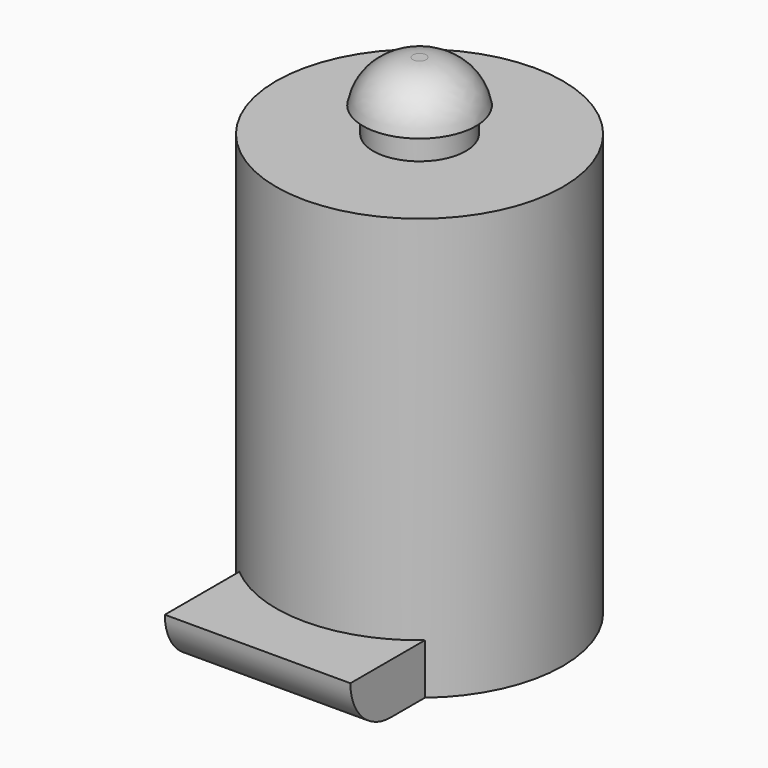
from build123d import *

# Parameters (mm, degrees)
F0_R      = 8.5
F0_R_2    = 6.5
F1_DEPTH  = 23
F2_R      = 8.5
F3_DEPTH  = 2
F5_DEPTH  = 3
F6_R      = 2.99999
F7_R      = 2.75
F8_DEPTH  = 1.5
F9_R      = 3.35
F10_DEPTH = 2.5


# Not quite as in the source:
# - a fillet or chamfer that OpenCascade refuses, or shapes differently, is made with other operations: its cross-section is extruded or revolved along the edge and cut away or added
# - a fillet or chamfer is up to 0.001 mm smaller than in the source, because OpenCascade refuses the exact size


with BuildPart() as f1:
    # F0 (on Top) → F1 (new body)
    with BuildSketch(Plane.XY):
        Circle(F0_R)
        Circle(F0_R_2, mode=Mode.SUBTRACT)
    extrude(amount=F1_DEPTH)

    # F2 (on face) → F3 (join)
    with BuildSketch(Plane.XY.offset(23)):
        Circle(F2_R)
    extrude(amount=F3_DEPTH)

    # F4 (on face) → F5 (join)
    with BuildSketch(Plane(origin=(0, 0, 0), x_dir=(1, 0, 0), z_dir=(0, 0, -1))):
        with BuildLine():
            ThreePointArc((-5.5, 6.4807406984), (-2.9294798227, 7.9792322919), (0, 8.5))
            Line((0, 8.5), (0, 12))
            Line((0, 12), (-5.5, 12))
            Line((-5.5, 12), (-5.5, 6.4807406984))
        make_face()
        with BuildLine():
            Line((0, 12), (0, 8.5))
            ThreePointArc((0, 8.5), (2.9294798227, 7.9792322919), (5.5, 6.4807406984))
            Line((5.5, 6.4807406984), (5.5, 12))
            Line((5.5, 12), (0, 12))
        make_face()
    extrude(amount=-F5_DEPTH)

    # F6 (radius 3 in the source; OpenCascade refuses exactly that, so slightly less here)
    f6_edges = [f1.edges().sort_by_distance(p)[0] for p in [
        (0, -12, 0),
    ]]
    fillet(f6_edges, radius=F6_R)

    # F7 (on face) → F8 (join)
    with BuildSketch(Plane.XY.offset(25)):
        Circle(F7_R)
    extrude(amount=F8_DEPTH)

    # F9 (on face) → F10 (join)
    with BuildSketch(Plane.XY.offset(26.5)):
        Circle(F9_R)
    extrude(amount=F10_DEPTH)

    # F11: fillet of radius 3 on 1 edges, made by hand

    # F11_s1 → F11_t2 (revolve, cut)
    with BuildSketch(Plane.XZ):
        with BuildLine():
            ThreePointArc((3.35, 26.5), (2.3284517816, 28.2912878475), (0.3919601084, 29))
            Line((0.3919601084, 29), (3.35, 29))
            Line((3.35, 29), (3.35, 26.5))
        make_face()
    revolve(axis=Axis((0, 0, 29), (0, 0, 1)), mode=Mode.SUBTRACT)


solid = f1.part
